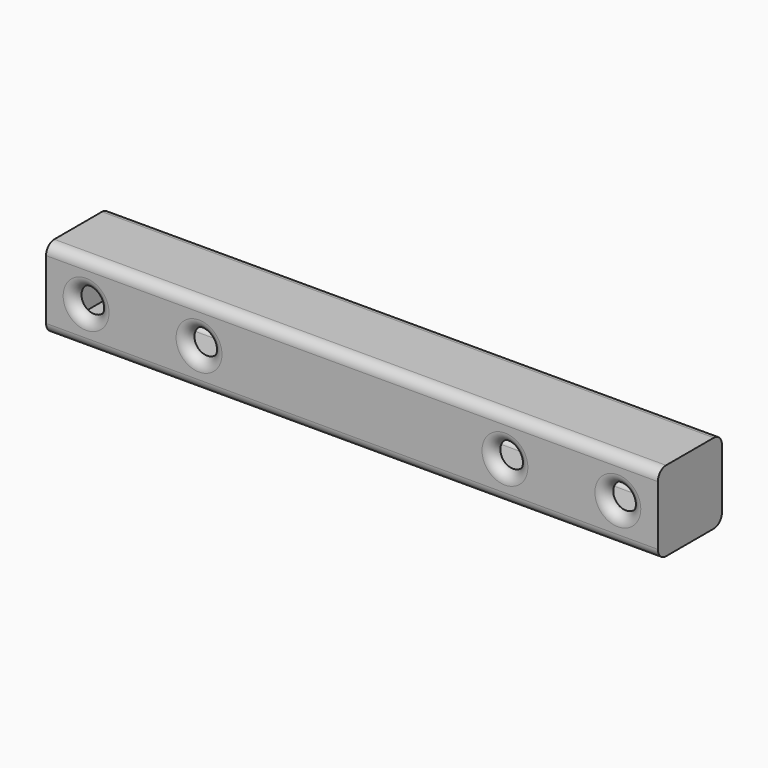
from build123d import *

# Parameters (mm, degrees)
F0_R     = 6.35
F1_DEPTH = 39.878
F2_R     = 5.08
F3_R     = 5.08
F4_T     = 2.54


# Not quite as in the source:
# - a shell that OpenCascade refuses in one call is made with other operations: the cavity is built on its own and cut out


with BuildPart() as f1:
    # F0 (on Front) → F1 (new body)
    with BuildSketch(Plane.XZ):
        Polygon((-112.522, -19.939), (152.4, -19.939), (152.4, 19.939), (76.2, 19.939), (0, 19.939), (-76.2, 19.939), (-112.522, 19.939), (-152.4, 19.939), (-152.4, -19.939), align=None)
        with Locations((-132.461, 0)):
            Circle(F0_R, mode=Mode.SUBTRACT)
        with Locations((-76.2, 0)):
            Circle(F0_R, mode=Mode.SUBTRACT)
        with Locations((76.2, 0)):
            Circle(F0_R, mode=Mode.SUBTRACT)
        with Locations((132.461, 0)):
            Circle(F0_R, mode=Mode.SUBTRACT)
    extrude(amount=F1_DEPTH)

    # F2
    f2_edges = [f1.edges().sort_by_distance(p)[0] for p in [
        (-138.811, -39.878, 0),
        (-82.55, -39.878, 0),
        (69.85, -39.878, 0),
    ]]
    fillet(f2_edges, radius=F2_R)

    # F3
    f3_edges = [f1.edges().sort_by_distance(p)[0] for p in [
        (126.111, -39.878, 0),
        (126.111, 0, 0),
        (69.85, 0, 0),
        (-82.55, 0, 0),
        (-138.811, 0, 0),
        (0, 0, -19.939),
        (0, 0, 19.939),
        (0, -39.878, 19.939),
        (0, -39.878, -19.939),
    ]]
    fillet(f3_edges, radius=F3_R)

    # F4: shell of thickness 2.54, made by hand


with BuildPart() as f4_core1:
    # F4_t2: copy of F1
    add(f1.part)

    # the walls: a layer under each face that stays
    f4_faces = [f4_core1.faces().sort_by_distance(p)[0] for p in [
        (0, -39.878, 0),
        (152.4, -19.939, 0),
        (0, -38.3901024484, -18.4511024484),
        (0, -38.3901024484, 18.4511024484),
        (-152.4, -19.939, 0),
        (-140.2988975516, -38.3901024484, 0),
        (-84.0378975516, -38.3901024484, 0),
        (68.3621024484, -38.3901024484, 0),
        (124.6231024484, -38.3901024484, 0),
        (0, -19.939, -19.939),
        (0, -1.4878975516, -18.4511024484),
        (0, 0, 0),
        (0, -1.4878975516, 18.4511024484),
        (0, -19.939, 19.939),
        (124.6231024484, -1.4878975516, 0),
        (68.3621024484, -1.4878975516, 0),
        (-84.0378975516, -1.4878975516, 0),
        (-140.2988975516, -1.4878975516, 0),
    ]]
    thicken(f4_faces, amount=-F4_T, mode=Mode.SUBTRACT)


with BuildPart() as f1_1:
    add(f1.part)

    # what is left inside the walls is the cavity
    f4_cavity = [f4_core1.part.solids().sort_by_distance(p)[0] for p in [
        (0, -24.892, -17.3736),
    ]]
    add(f4_cavity, mode=Mode.SUBTRACT)


solid = f1_1.part
